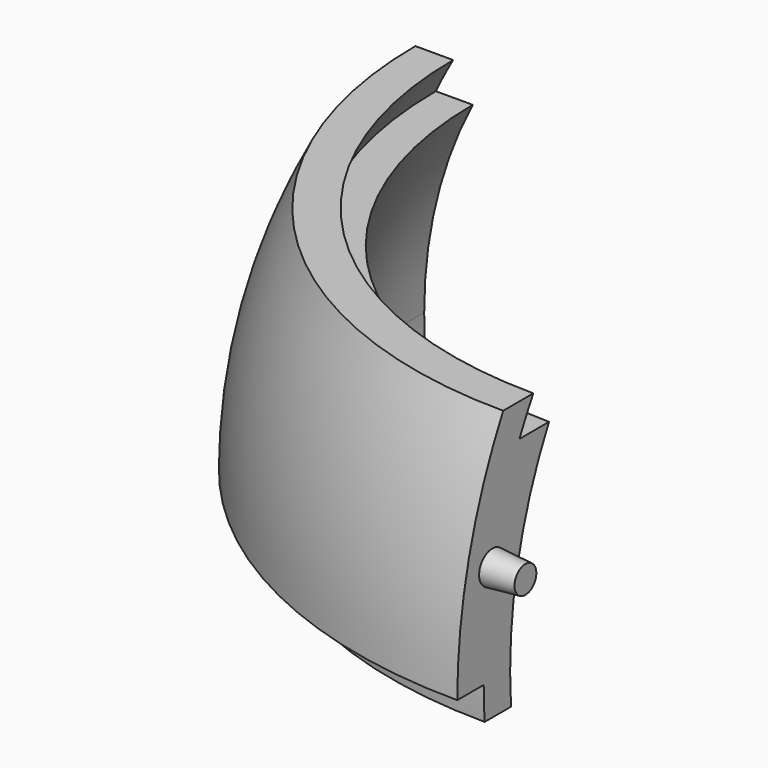
from build123d import *

# Parameters (mm, degrees)
F1_ANGLE = 90
F2_R     = 6.35
F3_DEPTH = 12.7
F3_TAPER = 5
F4_R     = 6.35
F5_DEPTH = 12.7
F5_TAPER = 5


# Not quite as in the source:
# - a feature names something its author has since deleted; it is built from what else it names


with BuildPart() as f1:
    # F0 (on Front) → F1 (revolve)
    with BuildSketch(Plane.XZ):
        with BuildLine():
            Line((-190.5, 0), (-177.7999999529, -0.0040913673))
            ThreePointArc((-177.7999999529, -0.0040913673), (-177.6863527462, -6.3561031883), (-177.3458485559, -12.7))
            Line((-177.3458485559, -12.7), (-164.6108137396, -12.7))
            ThreePointArc((-164.6108137396, -12.7), (-164.9776583118, -6.354703608), (-165.1, 1.06856e-05))
            ThreePointArc((-165.1, 1.06856e-05), (-160.3732216696, 39.2229495488), (-146.4635449523, 76.2))
            Line((-146.4635449523, 76.2), (-160.6437051366, 76.2))
            ThreePointArc((-160.6437051366, 76.2), (-157.4396201151, 82.6172259157), (-153.9793167929, 88.9))
            Line((-153.9793167929, 88.9), (-168.4845393501, 88.9))
            ThreePointArc((-168.4845393501, 88.9), (-184.9142432943, 45.792713688), (-190.5, 0))
        make_face()
    revolve(axis=Axis((0, 0, 38.1), (0, 0, 1)), revolution_arc=F1_ANGLE)

    # F2 (on face) → F3 (join)
    with BuildSketch(Plane.YZ):
        with Locations((-173.669888006, 38.1)):
            Circle(F2_R)
    extrude(amount=F3_DEPTH, taper=F3_TAPER)

    # F4 (on face) → F5 (cut)
    with BuildSketch(Plane(origin=(0, 0, 0), x_dir=(-1, 0, 0), z_dir=(0, 1, 0))):
        with Locations((173.669888006, 38.1)):
            Circle(F4_R)
    extrude(amount=-F5_DEPTH, taper=F5_TAPER, mode=Mode.SUBTRACT)


solid = f1.part
